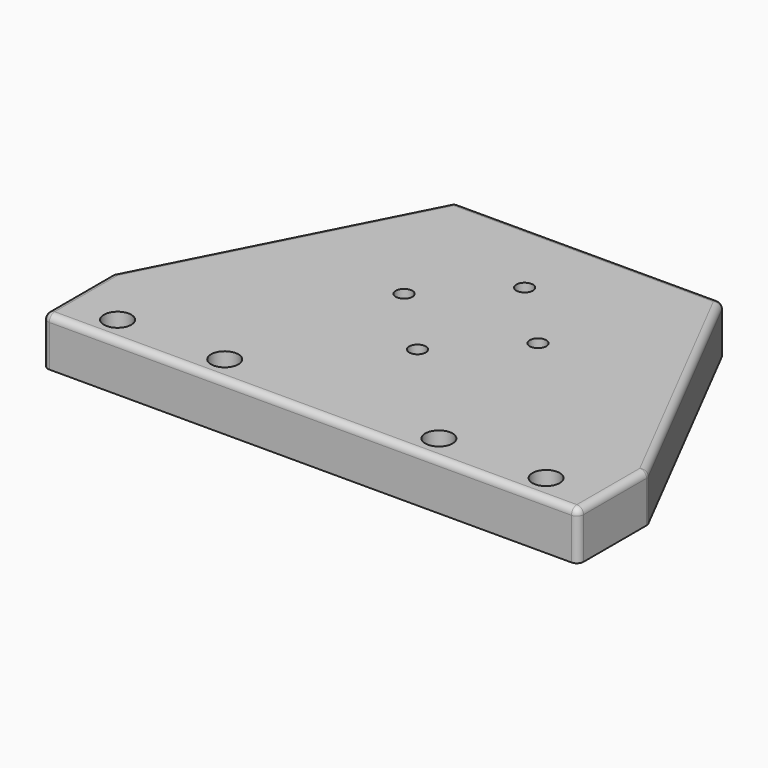
from build123d import *

# Parameters (mm, degrees)
F1_DEPTH       = 18
F2_D           = 6.2
F2_CBORE_D     = 10.2
F2_CBORE_DEPTH = 7
F4_D           = 6.2
F4_CBORE_D     = 10.2
F4_CBORE_DEPTH = 6.5
F5_R           = 2.5


with BuildPart() as f1:
    # F0 (on Top) → F1 (new body)
    with BuildSketch(Plane.XY):
        Polygon((-80, 0), (0, 0), (100, 0), (100, 32.5), (50, 130), (0, 130), (-50, 130), (-100, 32.5), (-100, 0), align=None)
    extrude(amount=F1_DEPTH)

    # F2 (through all)
    with Locations(Plane(origin=(0, 0, 0), x_dir=(1, 0, 0), z_dir=(0, 0, -1))):
        with Locations((0, -100), (25, -75), (0, -50), (-25, -75)):
            CounterBoreHole(F2_D / 2, F2_CBORE_D / 2, F2_CBORE_DEPTH)

    # F4 (through all)
    with Locations(Plane.XY.offset(18)):
        with Locations((-80, 10), (-40, 10), (40, 10), (80, 10)):
            CounterBoreHole(F4_D / 2, F4_CBORE_D / 2, F4_CBORE_DEPTH)

    # F5
    f5_edges = [f1.edges().sort_by_distance(p)[0] for p in [
        (-100, 32.5, 9),
        (-100, 16.25, 18),
        (0, 0, 18),
        (100, 16.25, 18),
        (-75, 81.25, 18),
        (75, 81.25, 18),
        (50, 130, 9),
        (-50, 130, 9),
        (100, 0, 9),
        (-100, 0, 9),
        (100, 32.5, 9),
        (0, 130, 18),
    ]]
    fillet(f5_edges, radius=F5_R)


solid = f1.part
